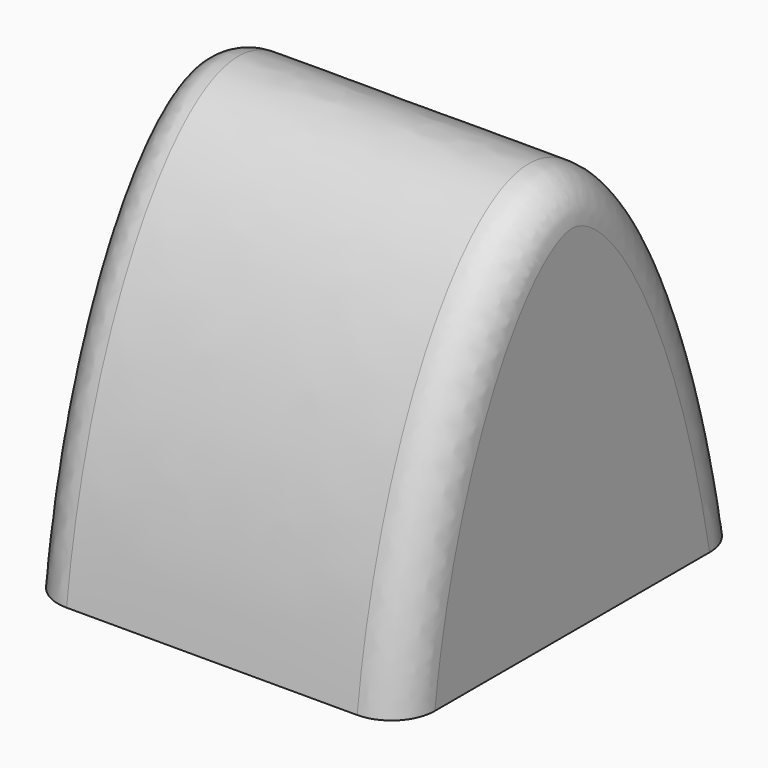
from build123d import *

# Parameters (mm, degrees)
F4_DEPTH = 35
F6_DEPTH = 33
F7_R     = 4


# Not quite as in the source:
# - a feature names something its author has since deleted; it is built from what else it names


with BuildPart() as f4:
    # F3 (on Right) → F4 (new body)
    with BuildSketch(Plane.YZ):
        with BuildLine():
            Line((-20, 0), (0, 0))
            Line((0, 0), (0, 37))
            add(Edge.make_bspline(
                [(0, 37), (-8.5256332532, 37.0518802553), (-17.6288448274, 20.054070279), (-20, 0)],
                knots=[0.5, 0.5, 0.5, 0.5, 1, 1, 1, 1], degree=3))
        make_face()
        with BuildLine():
            Line((0, 37), (0, 0))
            Line((0, 0), (20, 0))
            add(Edge.make_bspline(
                [(20, 0), (16.4736881852, 19.8465492576), (8.5256332532, 36.9481197447), (0, 37)],
                knots=[0, 0, 0, 0, 0.5, 0.5, 0.5, 0.5], degree=3))
        make_face()
    extrude(amount=F4_DEPTH)

    # F5 (on face) → F6 (cut)
    with BuildSketch(Plane(origin=(0, 0, 0), x_dir=(1, 0, 0), z_dir=(0, 0, -1))):
        Polygon((2, 2.4), (2, 0), (2, -2.4), (33, -2.4), (33, 0), (33, 2.4), align=None)
    extrude(amount=-F6_DEPTH, mode=Mode.SUBTRACT)

    # F7
    f7_edges = [f4.edges().sort_by_distance(p)[0] for p in [
        (35, -0.138558, 36.999345),
        (0, -0.138558, 36.999345),
    ]]
    fillet(f7_edges, radius=F7_R)


solid = f4.part
